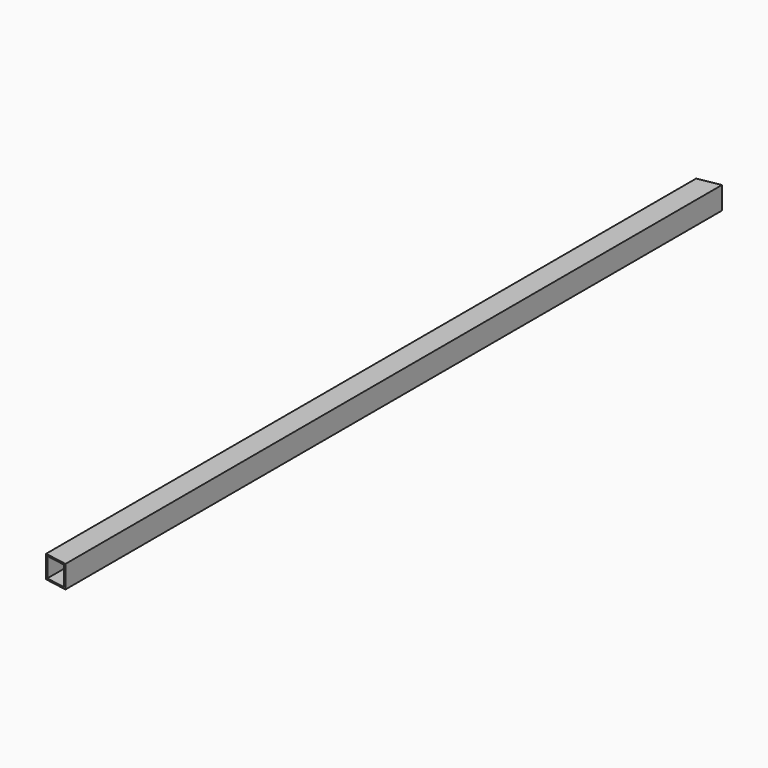
from build123d import *

# Parameters (mm, degrees)
F0_W     = 25.4
F0_H     = 25.4
F0_W_2   = 22.225
F0_H_2   = 22.225
F1_DEPTH = 462.28
F3_DEPTH = 25.401


# Not quite as in the source:
# - a pattern or mirror of a feature is missing from the dataset's text; its kind, count and spacing are read off the source's solid


with BuildPart() as f1:
    # F0 (on Front) → F1 (new body, symmetric)
    with BuildSketch(Plane.XZ):
        Rectangle(F0_W, F0_H)
        Rectangle(F0_W_2, F0_H_2, mode=Mode.SUBTRACT)
    extrude(amount=F1_DEPTH, both=True)

    # F2 (on face) → F3 (cut, through all)
    with BuildSketch(Plane.XY.offset(12.7)):
        Polygon((12.7, 462.28), (-12.7, 462.28), (-12.7, 457.80129469), align=None)
    f3 = extrude(amount=-F3_DEPTH, mode=Mode.SUBTRACT)

    # F3_copies: F3 across plane
    add(f3.mirror(Plane(origin=(0, 0, 0), x_dir=(0, 0, -1), z_dir=(0, -1, 0))), mode=Mode.SUBTRACT)


solid = f1.part
